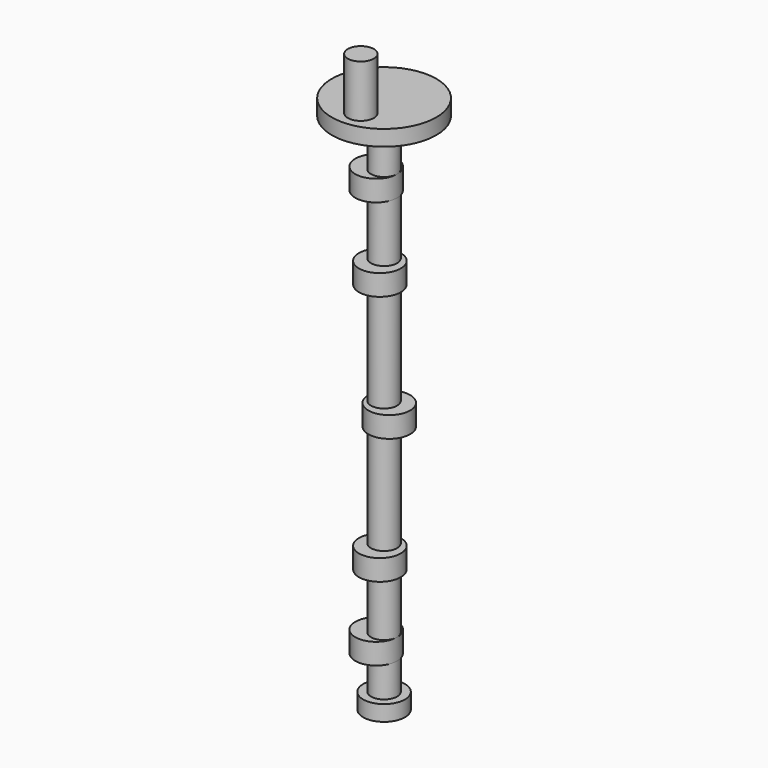
from build123d import *

# Parameters (mm, degrees)
F0_R          = 4
F1_DEPTH      = 3
F1_DEPTH_BACK = 1
F2_R          = 2.5
F3_DEPTH      = 98
F5_R          = 4
F6_DEPTH      = 4
F8_R          = 4
F9_DEPTH      = 4
F11_R         = 4
F12_DEPTH     = 4
F14_R         = 4
F15_DEPTH     = 4
F17_R         = 4
F18_DEPTH     = 4
F20_START     = 2
F19_R         = 10
F20_DEPTH     = 3
F21_R         = 2.5
F22_DEPTH     = 10
F24_R         = 2
F24_R_2       = 1
F25_DEPTH     = 1
F26_R         = 4
F26_R_2       = 2.5
F27_DEPTH     = 3


# Not quite as in the source:
# - a feature names something its author has since deleted; it is built from what else it names


with BuildPart() as f1:
    # F0 (on Top) → F1 (new body, two sides)
    with BuildSketch(Plane.XY) as f1_sk:
        Circle(F0_R)
    extrude(amount=F1_DEPTH)
    extrude(f1_sk.sketch, amount=-F1_DEPTH_BACK)

    # F2 (on Top) → F3 (join)
    with BuildSketch(Plane.XY):
        Circle(F2_R)
    extrude(amount=-F3_DEPTH)

    # F5 (on offset) → F6 (join)
    with BuildSketch(Plane.XY.offset(-50)):
        with Locations((1, 0)):
            Circle(F5_R)
    extrude(amount=F6_DEPTH)

    # F8 (on offset) → F9 (join)
    with BuildSketch(Plane.XY.offset(-26)):
        with Locations((0, -1)):
            Circle(F8_R)
    extrude(amount=F9_DEPTH)

    # F11 (on offset) → F12 (join)
    with BuildSketch(Plane.XY.offset(-11)):
        with Locations((-1.5, 0)):
            Circle(F11_R)
    extrude(amount=F12_DEPTH)

    # F14 (on offset) → F15 (join)
    with BuildSketch(Plane.XY.offset(-74)):
        with Locations((0, -1)):
            Circle(F14_R)
    extrude(amount=F15_DEPTH)

    # F17 (on offset) → F18 (join)
    with BuildSketch(Plane.XY.offset(-89)):
        with Locations((-1.5, 0)):
            Circle(F17_R)
    extrude(amount=F18_DEPTH)

    # F19 (on Top) → F20 (join)
    with BuildSketch(Plane.XY.offset(F20_START)):
        Circle(F19_R)
    extrude(amount=F20_DEPTH)

    # F21 (on face) → F22 (join)
    with BuildSketch(Plane.XY.offset(5)):
        with Locations((0.3544102503, -5.989523635)):
            Circle(F21_R)
    extrude(amount=F22_DEPTH)

    # F24 (on offset) → F25 (cut)
    with BuildSketch(Plane.XY.offset(-1)):
        Circle(F24_R)
        Circle(F24_R_2, mode=Mode.SUBTRACT)
    extrude(amount=-F25_DEPTH, mode=Mode.SUBTRACT)

    # F26 (on face) → F27 (join)
    with BuildSketch(Plane(origin=(0, 0, -98), x_dir=(1, 0, 0), z_dir=(0, 0, -1))):
        Circle(F26_R)
        Circle(F26_R_2, mode=Mode.SUBTRACT)
    extrude(amount=-F27_DEPTH)


solid = f1.part
